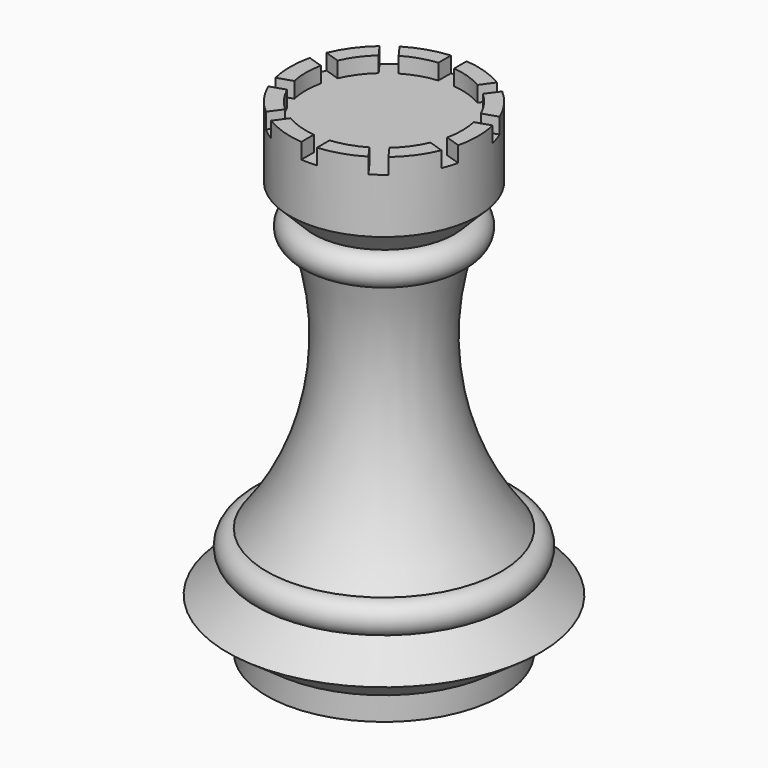
from build123d import *

# Parameters (mm, degrees)
F2_W            = 2.54
F2_H            = 2.54
F3_DEPTH        = 25.401
F3_DEPTH_BACK   = 25.401
F3_COPIES_COUNT = 5
F3_COPIES_ANGLE = 144


# Not quite as in the source:
# - a pattern or mirror of a feature is missing from the dataset's text; its kind, count and spacing are read off the source's solid


with BuildPart() as f1:
    # F0 (on Front) → F1 (revolve)
    with BuildSketch(Plane.XZ):
        with BuildLine():
            Line((0, 76.2), (0, 0))
            Line((0, 0), (19.05, 0))
            Line((19.05, 0), (19.05, 3.81))
            Line((19.05, 3.81), (25.4, 8.255))
            Line((25.4, 8.255), (19.05, 12.7))
            ThreePointArc((19.05, 12.7), (21.59, 15.24), (19.05, 17.78))
            ThreePointArc((19.05, 17.78), (10.2268710231, 37.1600383168), (11.43, 58.42))
            ThreePointArc((11.43, 58.42), (13.97, 60.96), (11.43, 63.5))
            Line((11.43, 63.5), (15.24, 67.31))
            Line((15.24, 67.31), (15.24, 78.74))
            Line((15.24, 78.74), (12.7, 78.74))
            Line((12.7, 78.74), (12.7, 76.2))
            Line((12.7, 76.2), (0, 76.2))
        make_face()
    revolve(axis=Axis((0, 0, 38.1), (0, 0, 1)))

    # F2 (on Front) → F3 (cut, two sides)
    with BuildSketch(Plane.XZ) as f3_sk:
        with Locations((0, 77.47)):
            Rectangle(F2_W, F2_H)
    f3 = extrude(amount=F3_DEPTH, mode=Mode.SUBTRACT) + extrude(f3_sk.sketch, amount=-F3_DEPTH_BACK, mode=Mode.SUBTRACT)

    # F3_copies: F3 ×5 about axis
    f3_copies_axis = Axis((0, 0, 0), (0, 0, 1))
    for i in range(1, F3_COPIES_COUNT):
        add(f3.rotate(f3_copies_axis, i * F3_COPIES_ANGLE / (F3_COPIES_COUNT - 1)), mode=Mode.SUBTRACT)


solid = f1.part
